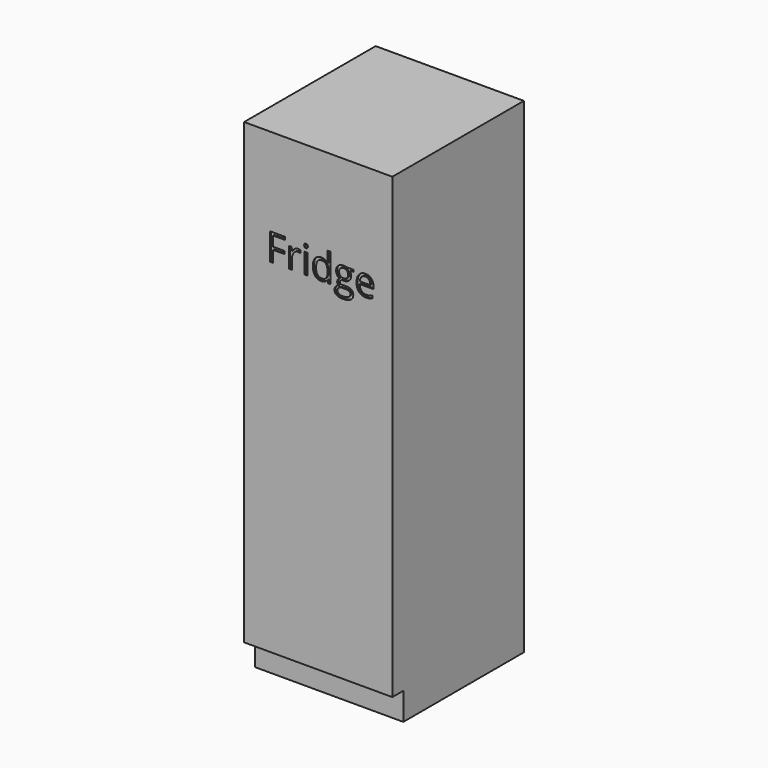
from build123d import *

# Parameters (mm, degrees)
F0_W         = 541
F0_H         = 1672
F1_DEPTH     = 600
F2_W         = 541
F2_H         = 100
F3_DEPTH     = 550
F4_TEXT_SIZE = 137.3832778791
F5_DEPTH     = 5


# Not quite as in the source:
# - Text() gives the source's letters only with a copy of the font that has no kerning and outlines rounded to 1/6400 em; it was checked with that copy


with BuildPart() as f1:
    # F0 (on Front) → F1 (new body)
    with BuildSketch(Plane.XZ):
        with Locations((-270.5, 836)):
            Rectangle(F0_W, F0_H)
    extrude(amount=F1_DEPTH)

    # F2 (on Front) → F3 (join)
    with BuildSketch(Plane.XZ):
        with Locations((-270.5, -50)):
            Rectangle(F2_W, F2_H)
    extrude(amount=F3_DEPTH)

    # F4 (on face) → F5 (cut)
    with BuildSketch(Plane.XZ.offset(600)):
        with Locations((-459.6321803921, 1253.6289511582)):
            Text('Fridge', F4_TEXT_SIZE, font='Open Sans', text_align=(TextAlign.LEFT, TextAlign.BOTTOM))
    extrude(amount=-F5_DEPTH, mode=Mode.SUBTRACT)


solid = f1.part
